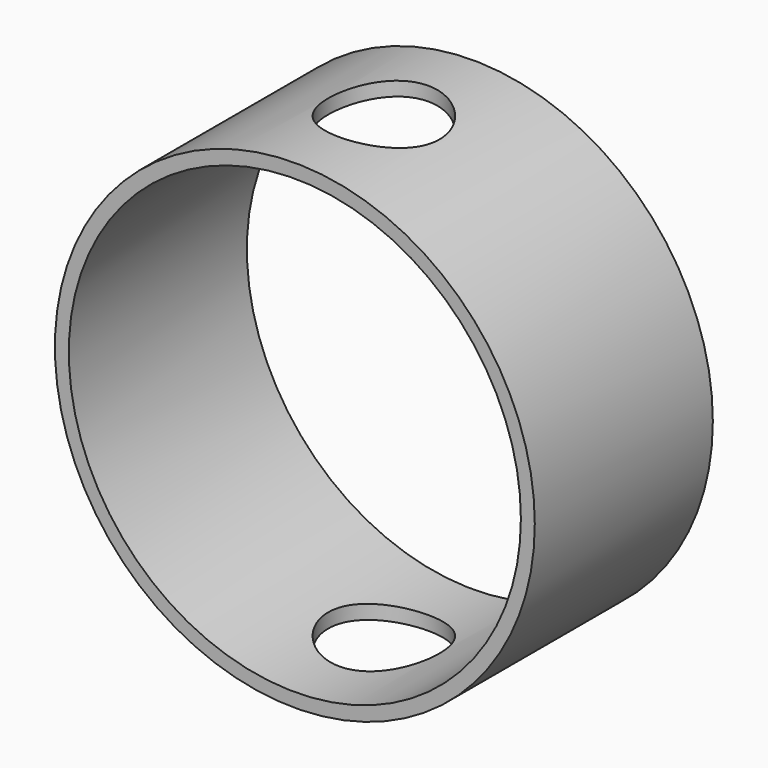
from build123d import *

# Parameters (mm, degrees)
F0_R          = 109.5375
F0_R_2        = 103.1875
F1_DEPTH      = 50.8
F1_DEPTH_BACK = 50.8
F3_R          = 25.4
F4_DEPTH      = 109.5385
F4_DEPTH_BACK = 109.5385


# Not quite as in the source:
# - a feature names something its author has since deleted; it is built from what else it names


with BuildPart() as f1:
    # F0 (on Front) → F1 (new body, two sides)
    with BuildSketch(Plane.XZ) as f1_sk:
        Circle(F0_R)
        Circle(F0_R_2, mode=Mode.SUBTRACT)
    extrude(amount=F1_DEPTH)
    extrude(f1_sk.sketch, amount=-F1_DEPTH_BACK)

    # F3 (on Top) → F4 (cut, two sides)
    with BuildSketch(Plane.XY) as f4_sk:
        Circle(F3_R)
    extrude(amount=-F4_DEPTH, mode=Mode.SUBTRACT)
    extrude(f4_sk.sketch, amount=F4_DEPTH_BACK, mode=Mode.SUBTRACT)


solid = f1.part
